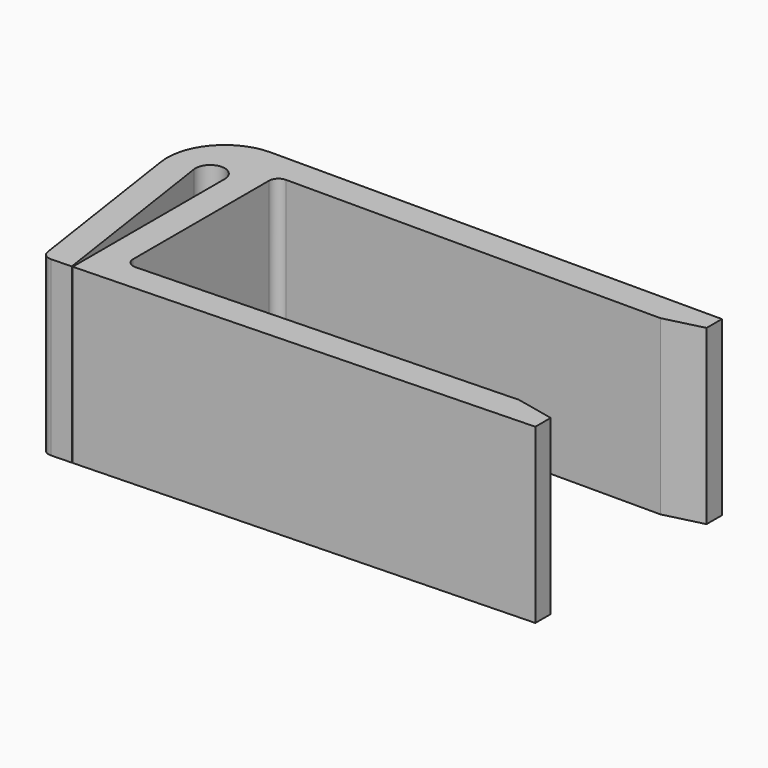
from build123d import *

# Parameters (mm, degrees)
F1_DEPTH      = 9
F1_DEPTH_BACK = 9
F3_DEPTH      = 9
F3_DEPTH_BACK = 9
F4_R          = 1
F5_R          = 1
F6_SIZE2      = 4
F6_SIZE       = 1
F7_SIZE2      = 4
F7_SIZE       = 1


# Not quite as in the source:
# - a feature names something its author has since deleted; it is built from what else it names


with BuildPart() as f1:
    # F0 (on Top) → F1 (new body, two sides)
    with BuildSketch(Plane.XY) as f1_sk:
        Polygon((0, 0), (44, 0), (44, 3), (-3, 3), (-3, -22.7954545455), (44, -21.3), (44, -18.3), (0, -19.7), align=None)
    extrude(amount=F1_DEPTH)
    extrude(f1_sk.sketch, amount=-F1_DEPTH_BACK)

    # F2 (on Top) → F3 (join, two sides)
    with BuildSketch(Plane.XY) as f3_sk:
        with BuildLine():
            ThreePointArc((-3, 3), (-7.5486403622, 0.9150686239), (-8.9383387138, -3.89178133))
            Line((-8.9383387138, -3.89178133), (-6.0984319756, -22.8940410174))
            Line((-6.0984319756, -22.8940410174), (-3.0999494186, -22.7986347542))
            Line((-3.0999494186, -22.7986347542), (-6.0252761047, -3.2248168493))
            ThreePointArc((-6.0252761047, -3.2248168493), (-4.6337098206, -1.4831910037), (-3, -3))
            Line((-3, -3), (-3, 3))
        make_face()
    extrude(amount=F3_DEPTH)
    extrude(f3_sk.sketch, amount=-F3_DEPTH_BACK)

    # F4
    f4_edges = [f1.edges().sort_by_distance(p)[0] for p in [
        (-3, 3, 0),
        (-6.098432, -22.894041, 0),
    ]]
    fillet(f4_edges, radius=F4_R)

    # F5
    f5_edges = [f1.edges().sort_by_distance(p)[0] for p in [
        (0, 0, 0),
        (0, -19.7, 0),
    ]]
    fillet(f5_edges, radius=F5_R)

    # F6
    f6_edges = [f1.edges().sort_by_distance(p)[0] for p in [
        (44, 0, 0),
    ]]
    f6_side = f1.faces().sort_by_distance((44, 1.5, 0))[0]
    chamfer(f6_edges, length=F6_SIZE, length2=F6_SIZE2, reference=f6_side)

    # F7
    f7_edges = [f1.edges().sort_by_distance(p)[0] for p in [
        (44, -18.3, 0),
    ]]
    f7_side = f1.faces().sort_by_distance((44, -19.8, 0))[0]
    chamfer(f7_edges, length=F7_SIZE, length2=F7_SIZE2, reference=f7_side)


solid = f1.part
